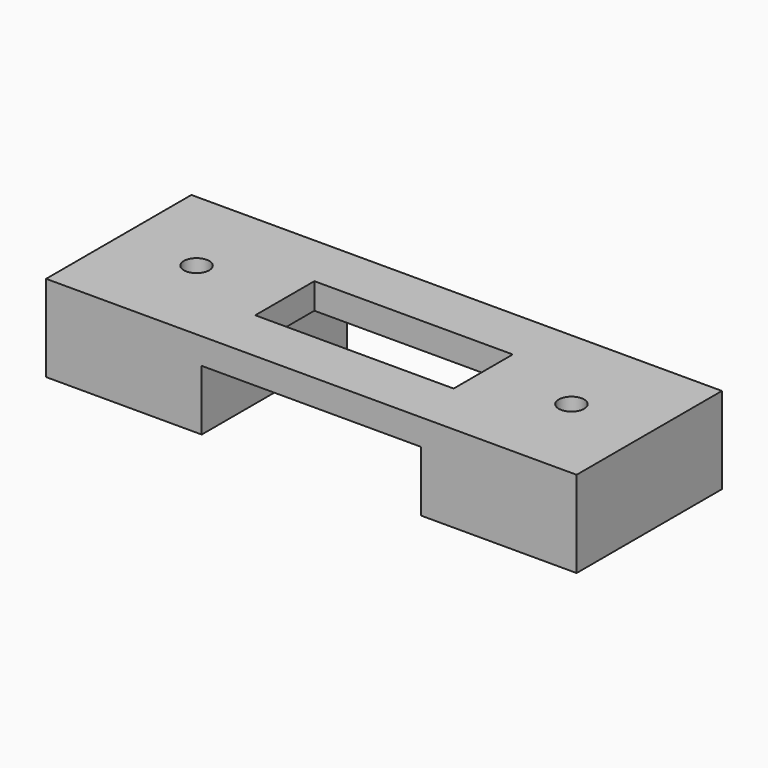
from build123d import *

# Parameters (mm, degrees)
F0_W      = 163.9416664839
F0_H      = 62.9752725363
F1_DEPTH  = 10
F2_DEPTH  = 20
F3_W      = 76.0346129537
F3_H      = 41.9552475214
F4_DEPTH  = 50
F5_DEPTH  = 10
F6_DEPTH  = 10
F7_DEPTH  = 10
F9_D      = 8.8
F11_D     = 8.8
F12_W     = 68.7855780125
F12_H     = 25.6147123873
F13_DEPTH = 25
F14_DEPTH = 10
F15_DEPTH = 10
F16_DEPTH = 5
F17_DEPTH = 5
F18_DEPTH = 15
F19_DEPTH = 5


with BuildPart() as f1:
    # F0 (on Top) → F1 (new body)
    with BuildSketch(Plane.XY):
        Rectangle(F0_W, F0_H)
    extrude(amount=F1_DEPTH)

    # F2 (add): a face of the model
    f2_faces = [f1.faces().sort_by_distance(p)[0] for p in [
        (0, 0, 10),
    ]]
    extrude(f2_faces, amount=F2_DEPTH)

    # F3 (on Front) → F4 (cut, symmetric)
    with BuildSketch(Plane.XZ):
        Rectangle(F3_W, F3_H)
    extrude(amount=F4_DEPTH, both=True, mode=Mode.SUBTRACT)

    # F5 (add): a face of the model
    f5_faces = [f1.faces().sort_by_distance(p)[0] for p in [
        (0, 0, 30),
    ]]
    extrude(f5_faces, amount=F5_DEPTH)

    # F6 (add): a face of the model
    f6_faces = [f1.faces().sort_by_distance(p)[0] for p in [
        (81.9708332419, 0, 20),
    ]]
    extrude(f6_faces, amount=F6_DEPTH)

    # F7 (add): a face of the model
    f7_faces = [f1.faces().sort_by_distance(p)[0] for p in [
        (-81.9708332419, 0, 20),
    ]]
    extrude(f7_faces, amount=F7_DEPTH)

    # F9 (through all)
    with Locations(Plane(origin=(0, 0, 0), x_dir=(1, 0, 0), z_dir=(0, 0, -1))):
        with Locations((-64.9940698594, 0)):
            Hole(F9_D / 2)

    # F11 (through all)
    with Locations(Plane(origin=(0, 0, 0), x_dir=(1, 0, 0), z_dir=(0, 0, -1))):
        with Locations((64.9940698594, 0)):
            Hole(F11_D / 2)

    # F12 (on face) → F13 (cut, symmetric)
    with BuildSketch(Plane(origin=(0, 0, 20.9776237607), x_dir=(1, 0, 0), z_dir=(0, 0, -1))):
        Rectangle(F12_W, F12_H)
    extrude(amount=F13_DEPTH, both=True, mode=Mode.SUBTRACT)

    # F14 (cut): a face of the model
    f14_faces = [f1.faces().sort_by_distance(p)[0] for p in [
        (-38.8465753115, 0, 0),
    ]]
    extrude(f14_faces, amount=-F14_DEPTH, mode=Mode.SUBTRACT)

    # F15 (cut): a face of the model
    f15_faces = [f1.faces().sort_by_distance(p)[0] for p in [
        (64.9940698594, -30.6583674335, 0),
    ]]
    extrude(f15_faces, amount=-F15_DEPTH, mode=Mode.SUBTRACT)

    # F16 (cut): a face of the model
    f16_faces = [f1.faces().sort_by_distance(p)[0] for p in [
        (64.9940698594, -30.6583674335, 10),
    ]]
    extrude(f16_faces, amount=-F16_DEPTH, mode=Mode.SUBTRACT)

    # F17 (cut): a face of the model
    f17_faces = [f1.faces().sort_by_distance(p)[0] for p in [
        (-38.8465753115, 0, 10),
    ]]
    extrude(f17_faces, amount=-F17_DEPTH, mode=Mode.SUBTRACT)

    # F18 (cut): a face of the model
    f18_faces = [f1.faces().sort_by_distance(p)[0] for p in [
        (37.0300300557, 0, 20.9776237607),
    ]]
    extrude(f18_faces, amount=-F18_DEPTH, mode=Mode.SUBTRACT)

    # F19 (add): a face of the model
    f19_faces = [f1.faces().sort_by_distance(p)[0] for p in [
        (0, 29.5434032158, 40),
    ]]
    extrude(f19_faces, amount=F19_DEPTH)


solid = f1.part
